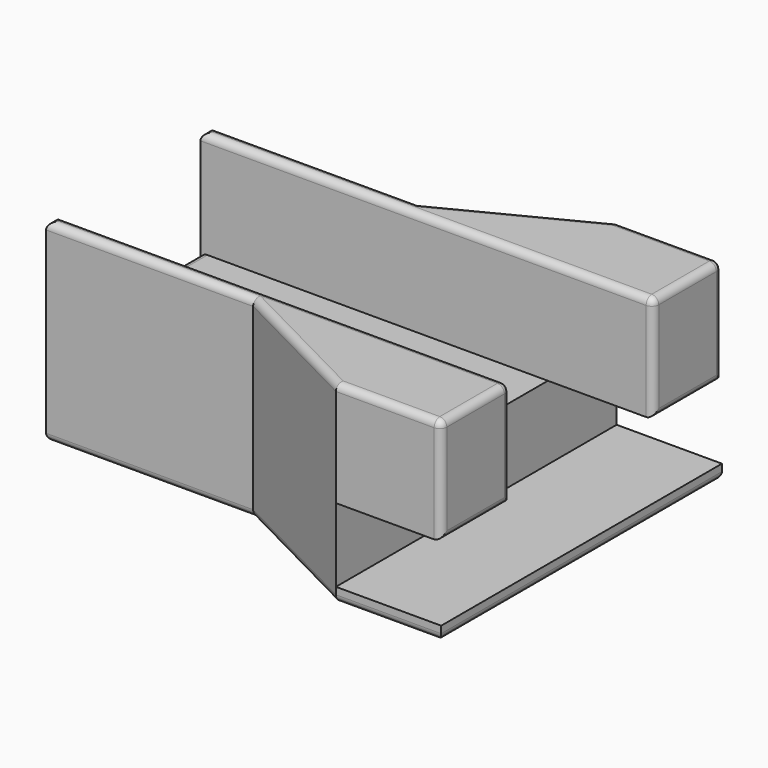
from build123d import *

# Parameters (mm, degrees)
F0_W     = 29.5
F0_H     = 12.75
F0_W_2   = 20
F0_W_3   = 15
F0_H_2   = 12.25
F1_DEPTH = 12.5
F2_DEPTH = 27.5
F4_DEPTH = 15
F6_R     = 0.99999


# Not quite as in the source:
# - a fillet or chamfer is up to 0.001 mm smaller than in the source, because OpenCascade refuses the exact size


with BuildPart() as f1:
    # F0 (on Top) → F1 (new body)
    with BuildSketch(Plane.XY):
        with Locations((-14.75, -6.375)):
            Rectangle(F0_W, F0_H)
        Polygon((20, -12.75), (0, -12.75), (-29.5, -12.75), (-29.5, -14.75), (0, -14.75), (20, -25), align=None)
        with Locations((10, -6.375)):
            Rectangle(F0_W_2, F0_H)
        with Locations((27.5, -6.375)):
            Rectangle(F0_W_3, F0_H)
        with Locations((27.5, -18.875)):
            Rectangle(F0_W_3, F0_H_2)
    extrude(amount=F1_DEPTH)

    # F0 (on Top) → F2 (join)
    with BuildSketch(Plane.XY):
        Polygon((20, -12.75), (0, -12.75), (-29.5, -12.75), (-29.5, -14.75), (0, -14.75), (20, -25), align=None)
        with Locations((27.5, -18.875)):
            Rectangle(F0_W_3, F0_H_2)
    extrude(amount=F2_DEPTH)

    # F3 (on face) → F4 (cut)
    with BuildSketch(Plane.YZ.offset(35)):
        Polygon((-25, 2), (0, 2), (0, 12.5), (-12.75, 12.5), (-25, 12.5), align=None)
    extrude(amount=-F4_DEPTH, mode=Mode.SUBTRACT)

    # F5: F1 across plane


with BuildPart() as f1_1:
    add(f1.part)
    add(f1.part.mirror(Plane.XZ))

    # F6 (radius 1 in the source; OpenCascade refuses exactly that, so slightly less here)
    f6_edges = [f1_1.edges().sort_by_distance(p)[0] for p in [
        (-14.75, -14.75, 0),
        (10, -19.875, 0),
        (27.5, -25, 0),
        (35, 0, 0),
        (27.5, 25, 0),
        (10, 19.875, 0),
        (-14.75, 14.75, 0),
        (-29.5, 0, 0),
        (-29.5, -13.75, 27.5),
        (-14.75, -14.75, 27.5),
        (10, -19.875, 27.5),
        (27.5, -25, 27.5),
        (35, -18.875, 27.5),
        (2.75, -12.75, 27.5),
        (-29.5, 13.75, 27.5),
        (-14.75, 14.75, 27.5),
        (10, 19.875, 27.5),
        (27.5, 25, 27.5),
        (35, 18.875, 27.5),
        (2.75, 12.75, 27.5),
        (35, 25, 20),
        (35, 18.875, 12.5),
        (35, 12.75, 20),
        (35, -18.875, 12.5),
        (35, -12.75, 20),
        (35, -25, 20),
        (-29.5, 0, 12.5),
    ]]
    fillet(f6_edges, radius=F6_R)


solid = f1_1.part
